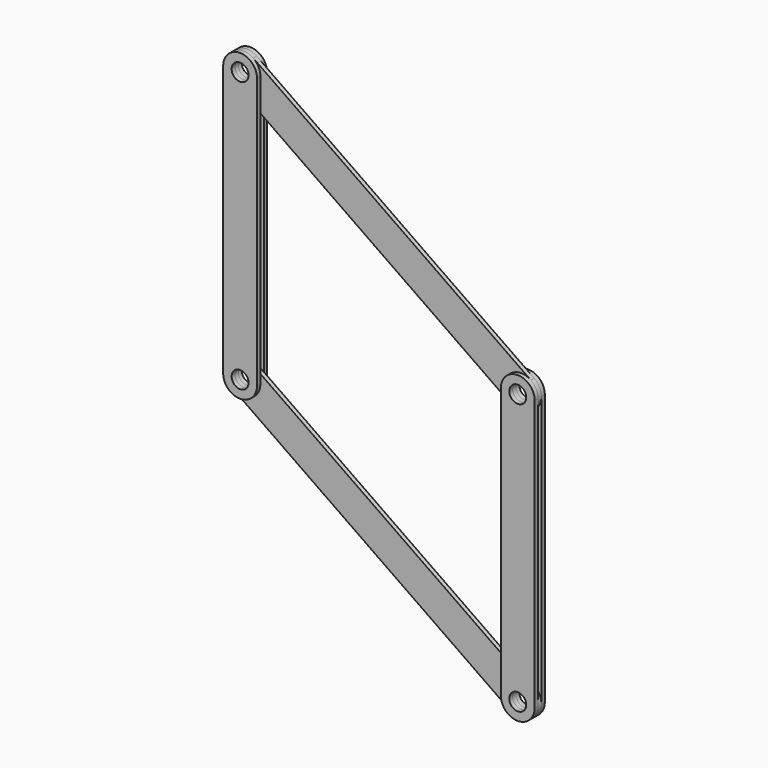
from build123d import *

# Parameters (mm, degrees)
F2_R     = 3.175
F3_DEPTH = 1.5875
F4_R     = 3.175
F5_DEPTH = 1.5875


# Not quite as in the source:
# - a variable given as a bare number and used for a length is read in inches; the dataset says mm whatever the document's units were


with BuildPart() as f3:
    # F2 (on Front) → F3 (new body)
    with BuildSketch(Plane.XZ):
        with BuildLine():
            Line((6.35, 0), (6.35, 101.6))
            ThreePointArc((6.35, 101.6), (0, 107.95), (-6.35, 101.6))
            Line((-6.35, 101.6), (-6.35, 0))
            ThreePointArc((-6.35, 0), (0, -6.35), (6.35, 0))
        make_face()
        Circle(F2_R, mode=Mode.SUBTRACT)
        with Locations((0, 101.6)):
            Circle(F2_R, mode=Mode.SUBTRACT)
    extrude(amount=F3_DEPTH)


with BuildPart() as f5:
    # F4 (on Front) → F5 (new body)
    with BuildSketch(Plane.XZ):
        with BuildLine():
            Line((107.8570888175, 34.2488983623), (3.6281274852, 106.8114480666))
            ThreePointArc((3.6281274852, 106.8114480666), (-5.2114480666, 105.2281274852), (-3.6281274852, 96.3885519334))
            Line((-3.6281274852, 96.3885519334), (100.6008338471, 23.8260022291))
            ThreePointArc((100.6008338471, 23.8260022291), (109.4404093989, 25.4093228105), (107.8570888175, 34.2488983623))
        make_face()
        with Locations((104.2289613323, 29.0374502957)):
            Circle(F4_R, mode=Mode.SUBTRACT)
        with Locations((0, 101.6)):
            Circle(F4_R, mode=Mode.SUBTRACT)
    extrude(amount=-F5_DEPTH)


with BuildPart() as f6_1:
    # F6: copy of F5
    add(f5.part.moved(Location((0, 0, -101.6))))


with BuildPart() as f7_1:
    # F7: copy of F3
    add(f3.part.moved(Location((104.2289613323, 0, -72.5625497043))))


with BuildPart() as f8_1:
    # F8: copy of F3
    add(f3.part.moved(Location((0, 3.175, 0))))


with BuildPart() as f8_2:
    # F8: copy of F7_1
    add(f7_1.part.moved(Location((0, 3.175, 0))))


solid = Compound([f3.part, f5.part, f6_1.part, f7_1.part, f8_1.part, f8_2.part])
